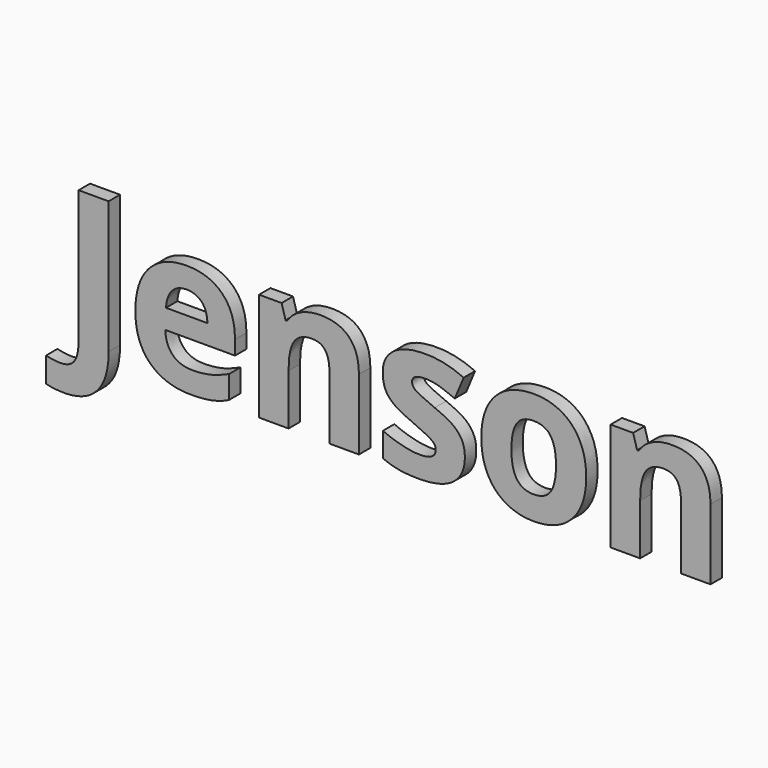
from build123d import *

# Parameters (mm, degrees)
F0_TEXT_SIZE = 83.3333333333
F1_DEPTH     = 6


# Not quite as in the source:
# - Text() gives the source's letters only with a copy of the font that has no kerning and outlines rounded to 1/6400 em; it was checked with that copy


with BuildPart() as f1:
    # F0 (on Front) → F1 (new body)
    with BuildSketch(Plane.XZ):
        with Locations((-284.7005208333, -114.8373750729)):
            Text('Jenson', F0_TEXT_SIZE, font='Open Sans', font_style=FontStyle.BOLD, text_align=(TextAlign.LEFT, TextAlign.BOTTOM))
    extrude(amount=F1_DEPTH)


solid = f1.part
